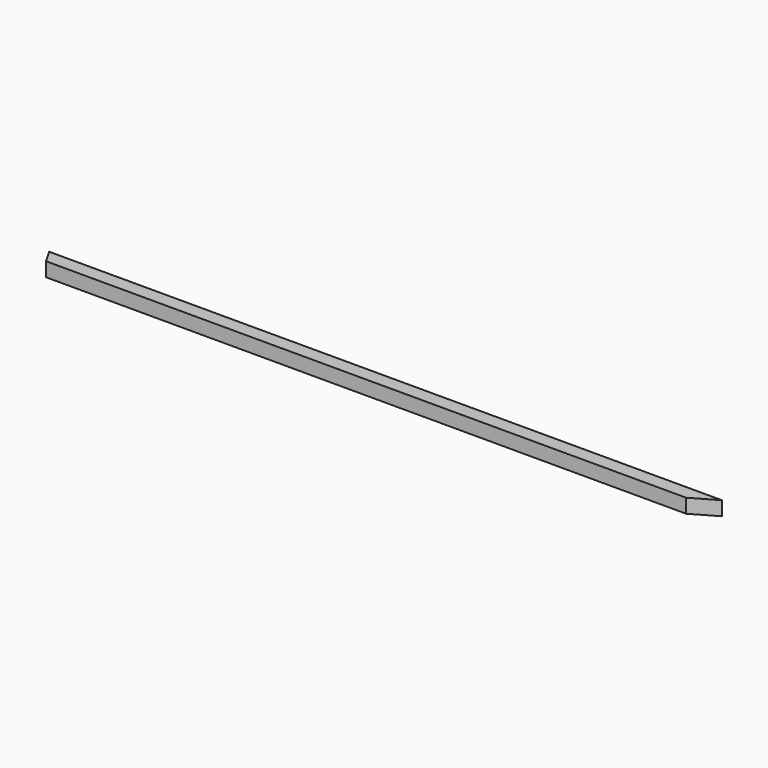
from build123d import *

# Parameters (mm, degrees)
F0_W        = 152.4
F0_H        = 3.175
F1_DEPTH    = 3.175
F2_T1_DEPTH = 23.6619672735
F3_T1_DEPTH = 35.0436157588


# Not quite as in the source:
# - a fillet or chamfer that OpenCascade refuses, or shapes differently, is made with other operations: its cross-section is extruded or revolved along the edge and cut away or added


with BuildPart() as f1:
    # F0 (on Front) → F1 (new body)
    with BuildSketch(Plane.XZ):
        with Locations((18.7120195478, 26.0135995823)):
            Rectangle(F0_W, F0_H)
    extrude(amount=F1_DEPTH)

    # F2: chamfer of 2.286 x 3.9594681461 on 1 edges, made by hand

    # F2_s2 → F2_t1 (cut)
    with BuildSketch(Plane.XY.offset(14.1826159455)):
        Polygon((-57.4879804522, 0.7844681461), (-55.2019804522, -3.175), (-57.4879804522, -3.175), align=None)
    extrude(amount=F2_T1_DEPTH, mode=Mode.SUBTRACT)

    # F3: chamfer of 3.556 x 6.1591726717 on 1 edges, made by hand

    # F3_s2 → F3_t1 (cut)
    with BuildSketch(Plane.XY.offset(8.4917917029)):
        Polygon((88.7528468761, -3.175), (94.9120195478, 0.381), (94.9120195478, -3.175), align=None)
    extrude(amount=F3_T1_DEPTH, mode=Mode.SUBTRACT)


solid = f1.part
